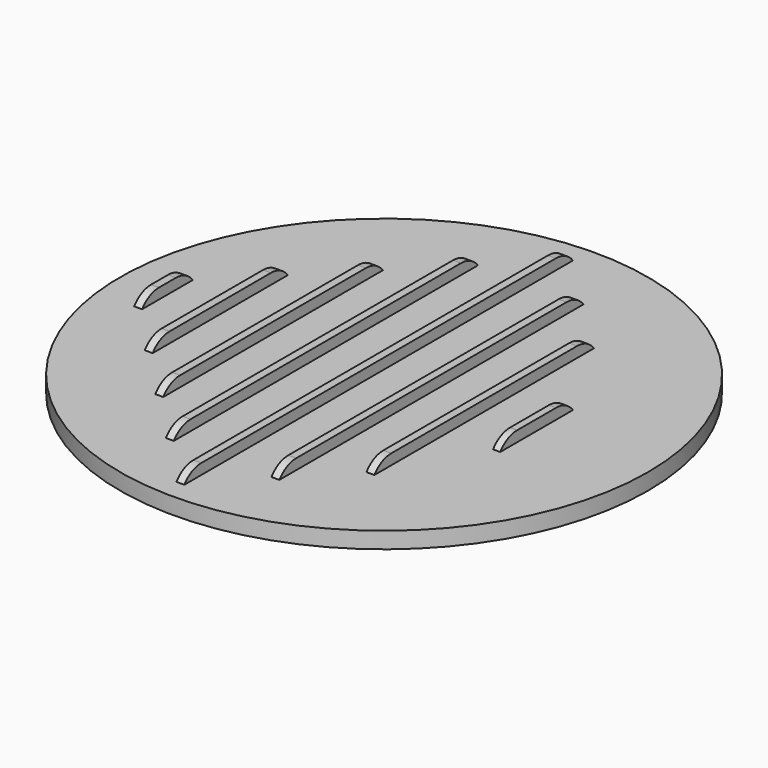
from build123d import *

# Parameters (mm, degrees)
F0_R         = 50
F1_DEPTH     = 3.1
F2_W         = 1.5
F2_H         = 92
F2_H_2       = 72
F2_H_3       = 52
F2_H_4       = 32
F2_H_5       = 12
F2_W_2       = 1.3582831621
F2_H_6       = 17.2204319388
F3_DEPTH     = 2
F4_T1_DEPTH  = 11.5
F4_T3_DEPTH  = 11.5
F4_T5_DEPTH  = 21.5
F4_T10_DEPTH = 21.5
F4_T15_DEPTH = 21.5
F4_T20_DEPTH = 21.5
F4_T25_DEPTH = 21.5
F4_T30_DEPTH = 21.5
F4_T35_DEPTH = 21.5
F4_T40_DEPTH = 21.5
F4_T45_DEPTH = 21.5
F4_T50_DEPTH = 21.3582831621
F4_T55_DEPTH = 21.3582831621


# Not quite as in the source:
# - a fillet or chamfer that OpenCascade refuses, or shapes differently, is made with other operations: its cross-section is extruded or revolved along the edge and cut away or added


with BuildPart() as f1:
    # F0 (on Top) → F1 (new body)
    with BuildSketch(Plane.XY):
        with Locations((1.7865982372, 0)):
            Circle(F0_R)
    extrude(amount=F1_DEPTH)

    # F2 (on face) → F3 (join)
    with BuildSketch(Plane.XY.offset(3.1)):
        Rectangle(F2_W, F2_H)
        with Locations((-10, 0)):
            Rectangle(F2_W, F2_H_2)
        with Locations((-20, 0)):
            Rectangle(F2_W, F2_H_3)
        with Locations((-30, 0)):
            Rectangle(F2_W, F2_H_4)
        with Locations((-40, 0)):
            Rectangle(F2_W, F2_H_5)
        with Locations((10, 0)):
            Rectangle(F2_W, F2_H_2)
        with Locations((20, 0)):
            Rectangle(F2_W, F2_H_3)
        with Locations((30, 0)):
            Rectangle(F2_W_2, F2_H_6)
    extrude(amount=F3_DEPTH)

    # F4: fillet of radius 5 on 16 edges, made by hand

    # F4_s2 → F4_t1 (cut)
    with BuildSketch(Plane.YZ.offset(9.25)):
        with BuildLine():
            ThreePointArc((-36, 3.1), (-34.2360679775, 4.572135955), (-32, 5.1))
            Line((-32, 5.1), (-36, 5.1))
            Line((-36, 5.1), (-36, 3.1))
        make_face()
        with BuildLine():
            ThreePointArc((36, 3.1), (34.2360679775, 4.572135955), (32, 5.1))
            Line((32, 5.1), (36, 5.1))
            Line((36, 5.1), (36, 3.1))
        make_face()
    extrude(amount=F4_T1_DEPTH, mode=Mode.SUBTRACT)

    # F4_s4 → F4_t3 (cut)
    with BuildSketch(Plane.YZ.offset(19.25)):
        with BuildLine():
            ThreePointArc((26, 3.1), (24.2360679775, 4.572135955), (22, 5.1))
            Line((22, 5.1), (26, 5.1))
            Line((26, 5.1), (26, 3.1))
        make_face()
        with BuildLine():
            ThreePointArc((-26, 3.1), (-24.2360679775, 4.572135955), (-22, 5.1))
            Line((-22, 5.1), (-26, 5.1))
            Line((-26, 5.1), (-26, 3.1))
        make_face()
    extrude(amount=F4_T3_DEPTH, mode=Mode.SUBTRACT)

    # F4_s6 → F4_t5 (cut)
    with BuildSketch(Plane.YZ.offset(-10.75)):
        with BuildLine():
            ThreePointArc((46, 3.1), (44.2360679775, 4.572135955), (42, 5.1))
            Line((42, 5.1), (46, 5.1))
            Line((46, 5.1), (46, 3.1))
        make_face()
        with BuildLine():
            ThreePointArc((-46, 3.1), (-44.2360679775, 4.572135955), (-42, 5.1))
            Line((-42, 5.1), (-46, 5.1))
            Line((-46, 5.1), (-46, 3.1))
        make_face()
    extrude(amount=F4_T5_DEPTH, mode=Mode.SUBTRACT)


with BuildPart() as f4_tool8:
    # F4_s9 → F4_t10 (new body)
    with BuildSketch(Plane.YZ.offset(0.75)):
        with BuildLine():
            ThreePointArc((36, 3.1), (34.2360679775, 4.572135955), (32, 5.1))
            Line((32, 5.1), (36, 5.1))
            Line((36, 5.1), (36, 3.1))
        make_face()
    extrude(amount=-F4_T10_DEPTH)

    split(bisect_by=Plane.YZ.offset(-0.75), keep=Keep.BOTTOM)


with BuildPart() as f1_1:
    add(f1.part)

    # F4_t7: cut F4_tool8
    add(f4_tool8.part, mode=Mode.SUBTRACT)


with BuildPart() as f4_tool13:
    # F4_s14 → F4_t15 (new body)
    with BuildSketch(Plane.YZ.offset(-9.25)):
        with BuildLine():
            ThreePointArc((26, 3.1), (24.2360679775, 4.572135955), (22, 5.1))
            Line((22, 5.1), (26, 5.1))
            Line((26, 5.1), (26, 3.1))
        make_face()
    extrude(amount=-F4_T15_DEPTH)

    split(bisect_by=Plane.YZ.offset(-10.75), keep=Keep.BOTTOM)


with BuildPart() as f1_2:
    add(f1_1.part)

    # F4_t12: cut F4_tool13
    add(f4_tool13.part, mode=Mode.SUBTRACT)


with BuildPart() as f4_tool18:
    # F4_s19 → F4_t20 (new body)
    with BuildSketch(Plane.YZ.offset(-19.25)):
        with BuildLine():
            ThreePointArc((16, 3.1), (14.2360679775, 4.572135955), (12, 5.1))
            Line((12, 5.1), (16, 5.1))
            Line((16, 5.1), (16, 3.1))
        make_face()
    extrude(amount=-F4_T20_DEPTH)

    split(bisect_by=Plane.YZ.offset(-20.75), keep=Keep.BOTTOM)


with BuildPart() as f1_3:
    add(f1_2.part)

    # F4_t17: cut F4_tool18
    add(f4_tool18.part, mode=Mode.SUBTRACT)


with BuildPart() as f4_tool23:
    # F4_s24 → F4_t25 (new body)
    with BuildSketch(Plane.YZ.offset(-29.25)):
        with BuildLine():
            ThreePointArc((6, 3.1), (4.2360679775, 4.572135955), (2, 5.1))
            Line((2, 5.1), (6, 5.1))
            Line((6, 5.1), (6, 3.1))
        make_face()
    extrude(amount=-F4_T25_DEPTH)

    split(bisect_by=Plane.YZ.offset(-30.75), keep=Keep.BOTTOM)


with BuildPart() as f1_4:
    add(f1_3.part)

    # F4_t22: cut F4_tool23
    add(f4_tool23.part, mode=Mode.SUBTRACT)


with BuildPart() as f4_tool28:
    # F4_s29 → F4_t30 (new body)
    with BuildSketch(Plane.YZ.offset(-50.75)):
        with BuildLine():
            ThreePointArc((-6, 3.1), (-4.2360679775, 4.572135955), (-2, 5.1))
            Line((-2, 5.1), (-6, 5.1))
            Line((-6, 5.1), (-6, 3.1))
        make_face()
    extrude(amount=F4_T30_DEPTH)

    split(bisect_by=Plane.YZ.offset(-30.75), keep=Keep.BOTTOM)


with BuildPart() as f1_5:
    add(f1_4.part)

    # F4_t27: cut F4_tool28
    add(f4_tool28.part, mode=Mode.SUBTRACT)


with BuildPart() as f4_tool33:
    # F4_s34 → F4_t35 (new body)
    with BuildSketch(Plane.YZ.offset(-40.75)):
        with BuildLine():
            ThreePointArc((-16, 3.1), (-14.2360679775, 4.572135955), (-12, 5.1))
            Line((-12, 5.1), (-16, 5.1))
            Line((-16, 5.1), (-16, 3.1))
        make_face()
    extrude(amount=F4_T35_DEPTH)

    split(bisect_by=Plane.YZ.offset(-20.75), keep=Keep.BOTTOM)


with BuildPart() as f1_6:
    add(f1_5.part)

    # F4_t32: cut F4_tool33
    add(f4_tool33.part, mode=Mode.SUBTRACT)


with BuildPart() as f4_tool38:
    # F4_s39 → F4_t40 (new body)
    with BuildSketch(Plane.YZ.offset(-30.75)):
        with BuildLine():
            ThreePointArc((-26, 3.1), (-24.2360679775, 4.572135955), (-22, 5.1))
            Line((-22, 5.1), (-26, 5.1))
            Line((-26, 5.1), (-26, 3.1))
        make_face()
    extrude(amount=F4_T40_DEPTH)

    split(bisect_by=Plane.YZ.offset(-10.75), keep=Keep.BOTTOM)


with BuildPart() as f1_7:
    add(f1_6.part)

    # F4_t37: cut F4_tool38
    add(f4_tool38.part, mode=Mode.SUBTRACT)


with BuildPart() as f4_tool43:
    # F4_s44 → F4_t45 (new body)
    with BuildSketch(Plane.YZ.offset(-20.75)):
        with BuildLine():
            ThreePointArc((-36, 3.1), (-34.2360679775, 4.572135955), (-32, 5.1))
            Line((-32, 5.1), (-36, 5.1))
            Line((-36, 5.1), (-36, 3.1))
        make_face()
    extrude(amount=F4_T45_DEPTH)

    split(bisect_by=Plane.YZ.offset(-0.75), keep=Keep.BOTTOM)


with BuildPart() as f1_8:
    add(f1_7.part)

    # F4_t42: cut F4_tool43
    add(f4_tool43.part, mode=Mode.SUBTRACT)


with BuildPart() as f4_tool48:
    # F4_s49 → F4_t50 (new body)
    with BuildSketch(Plane.YZ.offset(19.3208584189)):
        with BuildLine():
            ThreePointArc((-8.6102159694, 3.1), (-6.8462839469, 4.572135955), (-4.6102159694, 5.1))
            Line((-4.6102159694, 5.1), (-8.6102159694, 5.1))
            Line((-8.6102159694, 5.1), (-8.6102159694, 3.1))
        make_face()
    extrude(amount=F4_T50_DEPTH)

    split(bisect_by=Plane.YZ.offset(20.75), keep=Keep.TOP)


with BuildPart() as f1_9:
    add(f1_8.part)

    # F4_t47: cut F4_tool48
    add(f4_tool48.part, mode=Mode.SUBTRACT)


with BuildPart() as f4_tool53:
    # F4_s54 → F4_t55 (new body)
    with BuildSketch(Plane.YZ.offset(40.6791415811)):
        with BuildLine():
            ThreePointArc((8.6102159694, 3.1), (6.8462839469, 4.572135955), (4.6102159694, 5.1))
            Line((4.6102159694, 5.1), (8.6102159694, 5.1))
            Line((8.6102159694, 5.1), (8.6102159694, 3.1))
        make_face()
    extrude(amount=-F4_T55_DEPTH)

    split(bisect_by=Plane.YZ.offset(20.75), keep=Keep.TOP)


with BuildPart() as f1_10:
    add(f1_9.part)

    # F4_t52: cut F4_tool53
    add(f4_tool53.part, mode=Mode.SUBTRACT)


solid = f1_10.part
